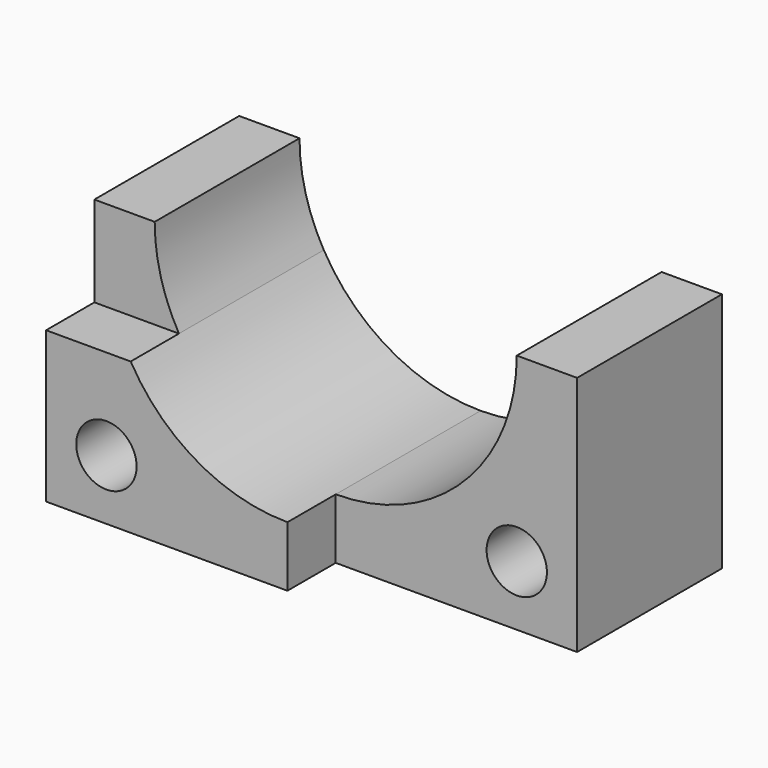
from build123d import *

# Parameters (mm, degrees)
F1_DEPTH = 30
F0_R     = 5
F2_DEPTH = 40


# Not quite as in the source:
# - a feature of the source that left no trace in its solid (it failed there, or was rolled back) is left out


with BuildPart() as f1:
    # F0 (on Front) → F1 (new body)
    with BuildSketch(Plane.XZ):
        with BuildLine():
            Line((10, 40), (0, 40))
            Line((0, 40), (0, 25))
            Line((0, 25), (14.0192378865, 25))
            ThreePointArc((14.0192378865, 25), (11.0222252113, 32.2354286469), (10, 40))
        make_face()
    extrude(amount=F1_DEPTH)



with BuildPart() as f1b:
    # F0 (on Front) → F1, piece 2 (new body)
    with BuildSketch(Plane.XZ):
        with BuildLine():
            Line((40, 10), (40, 0))
            Line((40, 0), (80, 0))
            Line((80, 0), (80, 40))
            Line((80, 40), (70, 40))
            ThreePointArc((70, 40), (61.2132034356, 18.7867965644), (40, 10))
        make_face()
        with Locations((70, 10)):
            Circle(F0_R, mode=Mode.SUBTRACT)
    extrude(amount=F1_DEPTH)


with BuildPart() as f1_1:
    add(f1.part)

    add(f1b.part)  # F2 merges F1b
    # F0 (on Front) → F2 (join)
    with BuildSketch(Plane.XZ):
        with BuildLine():
            Line((14.0192378865, 25), (0, 25))
            Line((0, 25), (0, 0))
            Line((0, 0), (40, 0))
            Line((40, 0), (40, 10))
            ThreePointArc((40, 10), (25, 14.0192378865), (14.0192378865, 25))
        make_face()
        with Locations((10, 10)):
            Circle(F0_R, mode=Mode.SUBTRACT)
    extrude(amount=F2_DEPTH)


solid = f1_1.part
